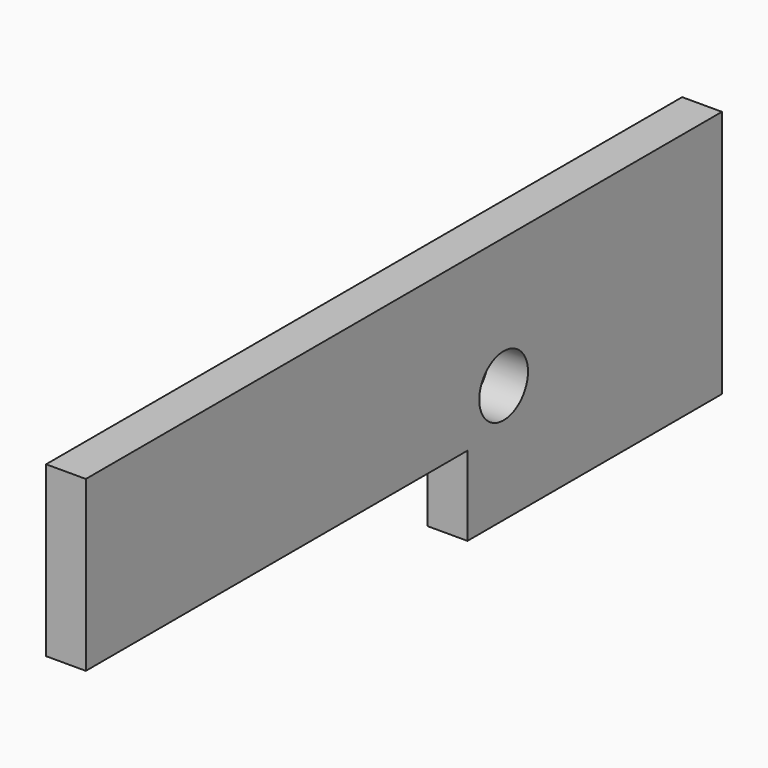
from build123d import *

# Parameters (mm, degrees)
F0_R     = 4.8652202412
F0_W     = 76.2
F0_H     = 12.7
F1_DEPTH = 6.35


# Not quite as in the source:
# - a length typed as a fraction of an inch, garbled in the dataset ("3 / 203.2 mm" for 3/8 in), is restored
# - a feature names something its author has since deleted; it is built from what else it names


with BuildPart() as f1:
    # F0 (on Right) → F1 (new body)
    with BuildSketch(Plane.YZ):
        Polygon((63.5, 7.14375), (-63.5, 7.14375), (-63.5, -7.14375), (12.7, -7.14375), (63.5, -7.14375), align=None)
        Polygon((63.5, -32.54375), (63.5, -7.14375), (12.7, -7.14375), (12.7, -19.84375), (12.7, -32.54375), align=None)
        with Locations((19.9129190296, -13.6523451656)):
            Circle(F0_R, mode=Mode.SUBTRACT)
        with Locations((-25.4, -13.49375)):
            Rectangle(F0_W, F0_H)
    extrude(amount=-F1_DEPTH)


solid = f1.part
